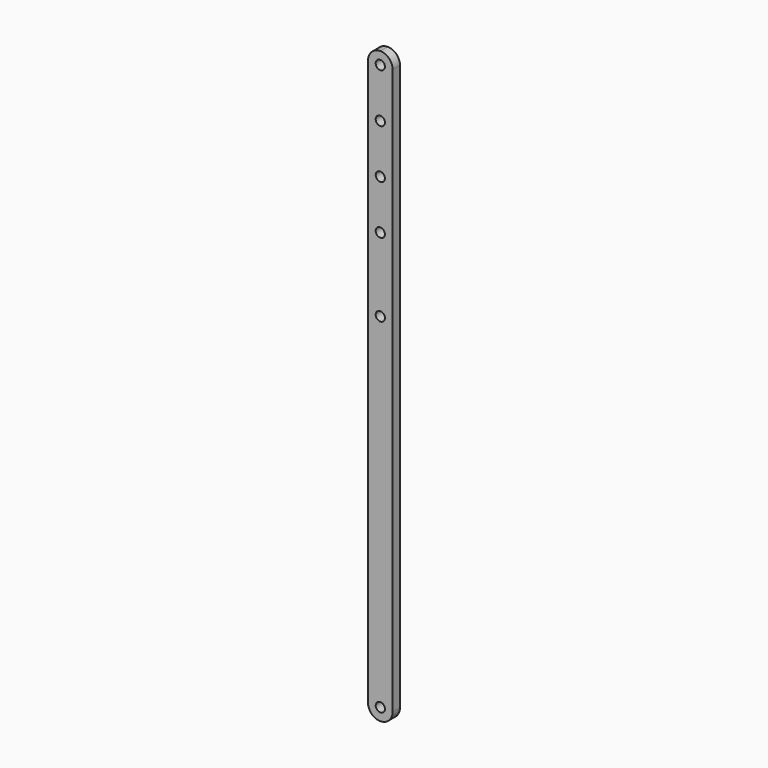
from build123d import *

# Parameters (mm, degrees)
F0_W     = 25.4
F0_H     = 609.6
F1_DEPTH = 4.7625
F2_R     = 12.69999
F4_D     = 9.525


# Not quite as in the source:
# - a fillet or chamfer is up to 0.001 mm smaller than in the source, because OpenCascade refuses the exact size


with BuildPart() as f1:
    # F0 (on Front) → F1 (new body, symmetric)
    with BuildSketch(Plane.XZ):
        Rectangle(F0_W, F0_H)
    extrude(amount=F1_DEPTH, both=True)

    # F2 (radius 12.7 in the source; OpenCascade refuses exactly that, so slightly less here)
    f2_edges = [f1.edges().sort_by_distance(p)[0] for p in [
        (12.7, 0, 304.8),
        (-12.7, 0, 304.8),
        (-12.7, 0, -304.8),
        (12.7, 0, -304.8),
    ]]
    fillet(f2_edges, radius=F2_R)

    # F4 (through all)
    with Locations(Plane.XZ.offset(4.7625)):
        with Locations((0, -292.1), (0, 292.1), (0, 63.5), (0, 241.3), (0, 190.5), (0, 139.7)):
            Hole(F4_D / 2)


solid = f1.part
